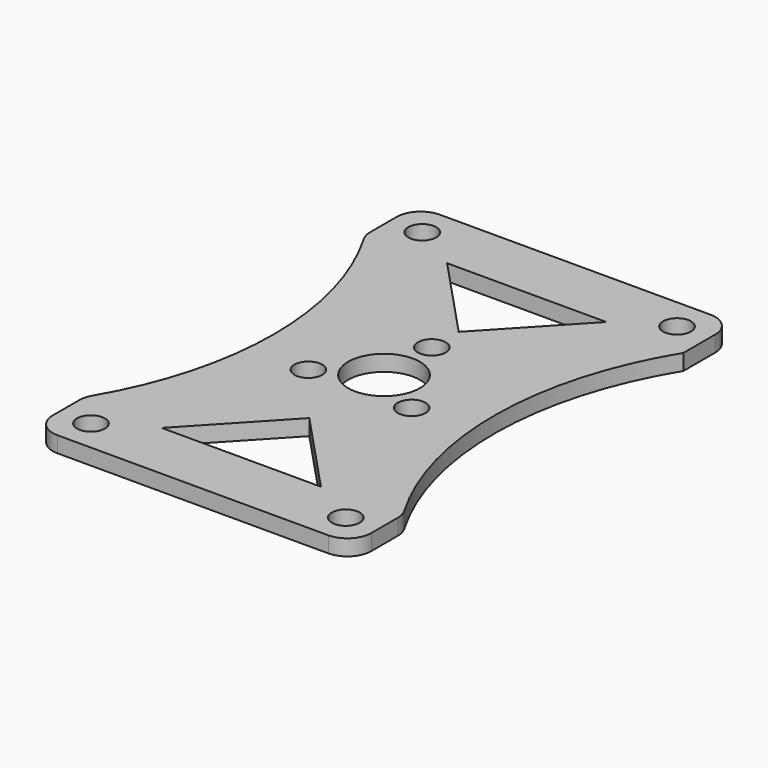
from build123d import *

# Parameters (mm, degrees)
F0_R     = 1.75
F0_R_2   = 4.5
F1_DEPTH = 2
F2_R     = 3


with BuildPart() as f1:
    # F0 (on Top) → F1 (new body)
    with BuildSketch(Plane.XY):
        with BuildLine():
            Line((20, 30), (-20, 30))
            Line((-20, 30), (-20, 22))
            ThreePointArc((-20, 22), (-13.8300253787, 0), (-20, -22))
            Line((-20, -22), (-20, -30))
            Line((-20, -30), (20, -30))
            Line((20, -30), (20, -22))
            ThreePointArc((20, -22), (13.8300253787, 0), (20, 22))
            Line((20, 22), (20, 30))
        make_face()
        with Locations((-16, -26)):
            Circle(F0_R, mode=Mode.SUBTRACT)
        with Locations((-6.4855394704, -3.7666666667)):
            Circle(F0_R, mode=Mode.SUBTRACT)
        Polygon((10, -22.4003139883), (0, -22.4003139883), (-10, -22.4003139883), (0, -11.7255505174), align=None, mode=Mode.SUBTRACT)
        with Locations((16, -26)):
            Circle(F0_R, mode=Mode.SUBTRACT)
        with Locations((6.4855394704, -3.7666666667)):
            Circle(F0_R, mode=Mode.SUBTRACT)
        with Locations((-16, 26)):
            Circle(F0_R, mode=Mode.SUBTRACT)
        Circle(F0_R_2, mode=Mode.SUBTRACT)
        with Locations((0, 7.5)):
            Circle(F0_R, mode=Mode.SUBTRACT)
        Polygon((0, 22.4003139883), (10, 22.4003139883), (0, 11.7255505174), (-10, 22.4003139883), align=None, mode=Mode.SUBTRACT)
        with Locations((16, 26)):
            Circle(F0_R, mode=Mode.SUBTRACT)
    extrude(amount=F1_DEPTH)

    # F2
    f2_edges = [f1.edges().sort_by_distance(p)[0] for p in [
        (-20, 30, 1),
        (-20, -30, 1),
        (20, -30, 1),
        (20, 30, 1),
        (20, -22, 1),
        (-20, -22, 1),
        (-20, 22, 1),
    ]]
    fillet(f2_edges, radius=F2_R)


solid = f1.part
